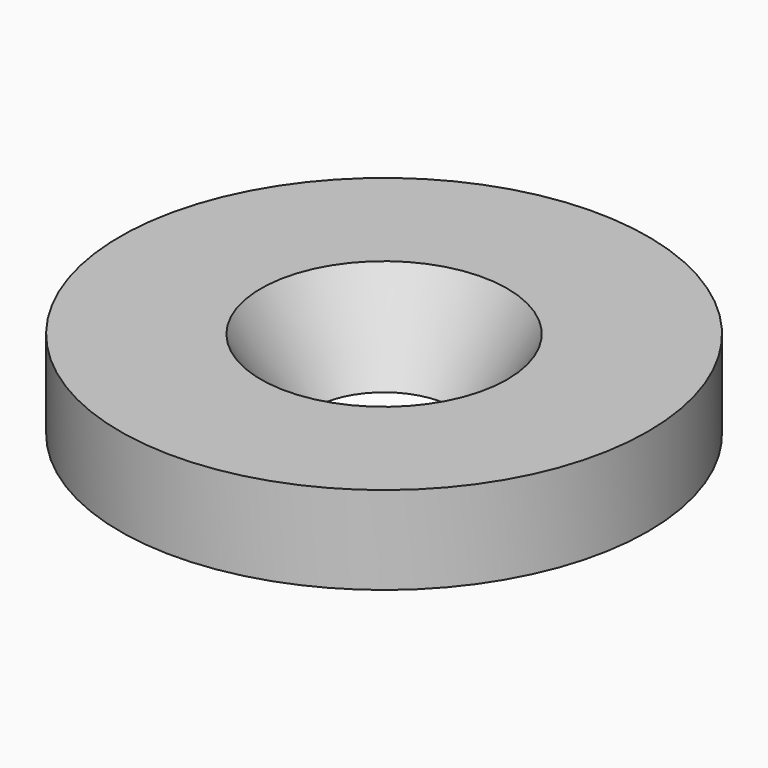
from build123d import *

# Parameters (mm, degrees)
F0_R     = 15
F0_R_2   = 4
F1_DEPTH = 5
F2_SIZE2 = 2.99999
F2_SIZE  = 4.99999


# Not quite as in the source:
# - a fillet or chamfer is up to 0.001 mm smaller than in the source, because OpenCascade refuses the exact size


with BuildPart() as f1:
    # F0 (on Top) → F1 (new body)
    with BuildSketch(Plane.XY):
        Circle(F0_R)
        Circle(F0_R_2, mode=Mode.SUBTRACT)
    extrude(amount=F1_DEPTH)

    # F2 (size 5 and 3 in the source; OpenCascade refuses exactly that, so slightly less here)
    f2_edges = [f1.edges().sort_by_distance(p)[0] for p in [
        (-4, 0, 5),
    ]]
    f2_side = f1.faces().sort_by_distance((-4, 0, 2.5))[0]
    chamfer(f2_edges, length=F2_SIZE, length2=F2_SIZE2, reference=f2_side)


solid = f1.part
